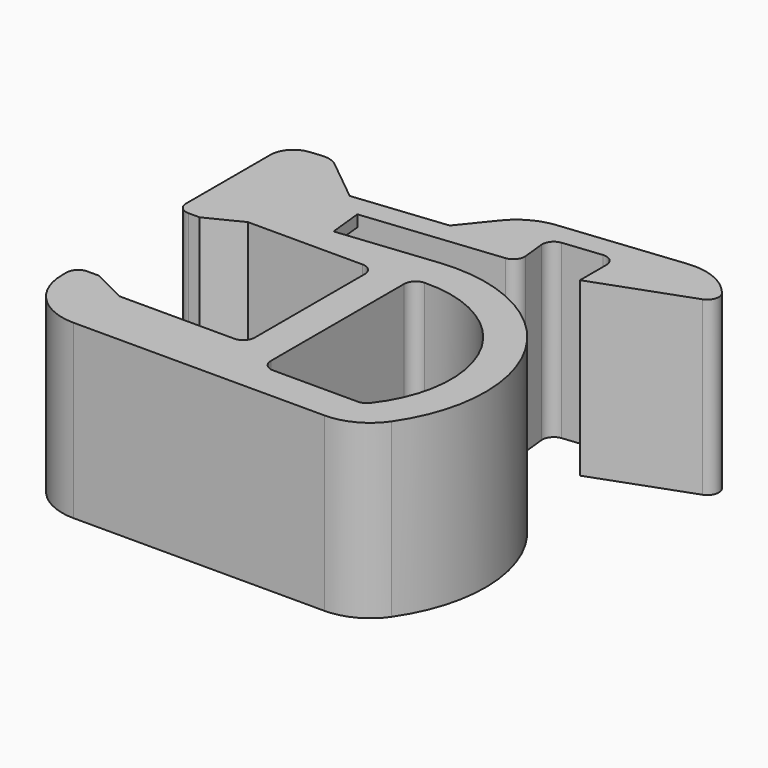
from build123d import *

# Parameters (mm, degrees)
F1_DEPTH    = 7.5
F2_T1_DEPTH = 40.8093190584
F2_T3_DEPTH = 25.3553390593
F2_T5_DEPTH = 40
F2_T7_DEPTH = 29.3169174454
F3_R        = 1
F5_DEPTH    = 1
F7_R        = 2


# Not quite as in the source:
# - a fillet or chamfer that OpenCascade refuses, or shapes differently, is made with other operations: its cross-section is extruded or revolved along the edge and cut away or added


with BuildPart() as f1:
    # F0 (on Top) → F1 (new body, symmetric)
    with BuildSketch(Plane.XY):
        with BuildLine():
            Line((12, 11.4339222498), (12, 7.4339222498))
            Line((12, 7.4339222498), (21.3969262079, 10.8541236831))
            Line((21.3969262079, 10.8541236831), (21.3969262079, 14.4325955519))
            Line((21.3969262079, 14.4325955519), (3.5841766184, 12.5604001283))
            Line((3.5841766184, 12.5604001283), (0.0437047985, 8.1882815452))
            Line((0.0437047985, 8.1882815452), (-8, 7.3428541036))
            Line((-8, 7.3428541036), (-12.3721185831, 10.8833259234))
            Line((-12.3721185831, 10.8833259234), (-16, 10.5020202215))
            Line((-16, 10.5020202215), (-16, -1.5))
            Line((-16, -1.5), (-14, -1.5))
            Line((-14, -1.5), (-11, 0))
            Line((-11, 0), (0, 0))
            Line((0, 0), (0, -14))
            Line((0, -14), (-11, -14))
            Line((-11, -14), (-14, -12.5))
            Line((-14, -12.5), (-16, -12.5))
            Line((-16, -12.5), (-16, -19))
            Line((-16, -19), (13.1190956366, -19))
            ThreePointArc((13.1190956366, -19), (16.1198863152, -4.0924328046), (2.9233065352, 3.4633984857))
            Line((2.9233065352, 3.4633984857), (-11, 2))
            Line((-11, 2), (-11, 5.0165248387))
            Line((-11, 5.0165248387), (7, 6.9084010735))
            Line((7, 6.9084010735), (6.5841766184, 10.8646962749))
            Line((6.5841766184, 10.8646962749), (12, 11.4339222498))
        make_face()
        with BuildLine():
            ThreePointArc((3, 0.4520743715), (13.0884587778, -4.7273070645), (11.8517750862, -16))
            Line((11.8517750862, -16), (3, -16))
            Line((3, -16), (3, 0.4520743715))
        make_face(mode=Mode.SUBTRACT)
    extrude(amount=F1_DEPTH, both=True)

    # F2: fillet of radius 5 on 4 edges, made by hand

    # F2_s2 → F2_t1 (cut)
    with BuildSketch(Plane.XY.offset(-20.4046595292)):
        with BuildLine():
            ThreePointArc((16.2633396262, 13.89303386), (19.3329992123, 13.2230634603), (21.3969262079, 10.8541236831))
            Line((21.3969262079, 10.8541236831), (21.3969262079, 14.4325955519))
            Line((21.3969262079, 14.4325955519), (16.2633396262, 13.89303386))
        make_face()
    extrude(amount=F2_T1_DEPTH, mode=Mode.SUBTRACT)

    # F2_s4 → F2_t3 (cut)
    with BuildSketch(Plane.XY.offset(-12.6776695297)):
        with BuildLine():
            ThreePointArc((2.2808114131, 10.9508781424), (3.7807474191, 12.1983617504), (5.6438989041, 12.776885664))
            Line((5.6438989041, 12.776885664), (3.5841766184, 12.5604001283))
            Line((3.5841766184, 12.5604001283), (2.2808114131, 10.9508781424))
        make_face()
    extrude(amount=F2_T3_DEPTH, mode=Mode.SUBTRACT)

    # F2_s6 → F2_t5 (cut)
    with BuildSketch(Plane.XY.offset(-20)):
        with BuildLine():
            ThreePointArc((-11, -19), (-14.5355339059, -17.5355339059), (-16, -14))
            Line((-16, -14), (-16, -19))
            Line((-16, -19), (-11, -19))
        make_face()
    extrude(amount=F2_T5_DEPTH, mode=Mode.SUBTRACT)

    # F2_s8 → F2_t7 (cut)
    with BuildSketch(Plane.XY.offset(-14.6584587227)):
        with BuildLine():
            ThreePointArc((14.9920579896, -16.8341336537), (13.1998162834, -18.4255320736), (10.8728728234, -19))
            Line((10.8728728234, -19), (13.1190956366, -19))
            ThreePointArc((13.1190956366, -19), (14.115390519, -17.9687915418), (14.9920579896, -16.8341336537))
        make_face()
    extrude(amount=F2_T7_DEPTH, mode=Mode.SUBTRACT)

    # F3
    f3_edges = [f1.edges().sort_by_distance(p)[0] for p in [
        (21.396926, 10.854124, 0),
        (7, 6.908401, 0),
        (-11, 5.016525, 0),
        (-11, 2, 0),
        (12, 11.433922, 0),
        (6.584177, 10.864696, 0),
        (0, 0, 0),
        (0, -14, 0),
        (11.851775, -16, 0),
        (3, -16, 0),
        (3, 0.452074, 0),
        (-16, -12.5, 0),
        (-16, -1.5, 0),
    ]]
    fillet(f3_edges, radius=F3_R)

    # F4 (on face) → F5 (join)
    with BuildSketch(Plane.XY.offset(7.5)):
        with BuildLine():
            Line((-5.9013941166, 5.552409911), (-10.1045284633, 5.1106426898))
            ThreePointArc((-10.1045284633, 5.1106426898), (-10.7431448255, 4.7852514008), (-11, 4.1161207944))
            Line((-11, 4.1161207944), (-11, 3.1106125148))
            ThreePointArc((-11, 3.1106125148), (-10.6691306064, 2.3674676894), (-9.8954715367, 2.1160906195))
            Line((-9.8954715367, 2.1160906195), (-5.5878087268, 2.5688442249))
            Line((-5.5878087268, 2.5688442249), (-5.9013941166, 5.552409911))
        make_face()
    extrude(amount=-F5_DEPTH)

    # F6: F1 across plane


with BuildPart() as f1_1:
    add(f1.part)
    add(f1.part.mirror(Plane.XY))

    # F7
    f7_edges = [f1_1.edges().sort_by_distance(p)[0] for p in [
        (-12.372119, 10.883326, 0),
        (-16, 10.50202, 0),
    ]]
    fillet(f7_edges, radius=F7_R)


solid = f1_1.part
